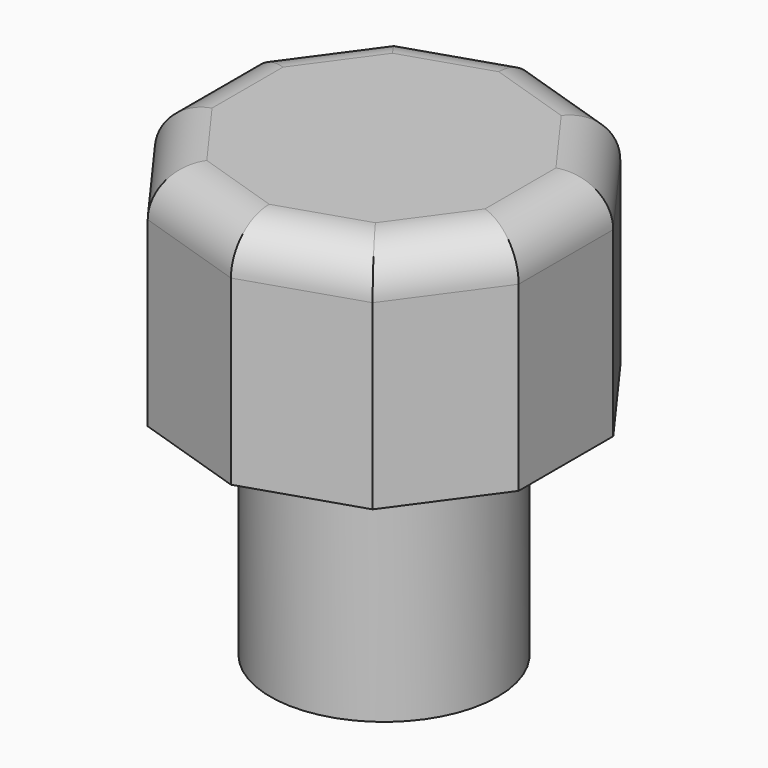
from build123d import *

# Parameters (mm, degrees)
F0_R     = 5
F0_R_2   = 1.6
F1_DEPTH = 10
F3_DEPTH = 8
F5_DEPTH = 2
F6_R     = 1.99999
F8_DEPTH = 3


# Not quite as in the source:
# - a fillet or chamfer is up to 0.001 mm smaller than in the source, because OpenCascade refuses the exact size


with BuildPart() as f1:
    # F0 (on Top) → F1 (new body)
    with BuildSketch(Plane.XY):
        Circle(F0_R)
        Circle(F0_R_2, mode=Mode.SUBTRACT)
    extrude(amount=F1_DEPTH)

    # F2 (on face) → F3 (join)
    with BuildSketch(Plane.XY.offset(10)):
        Polygon((8, -2.5993575699), (8, 2.5993575699), (4.94427191, 6.8052064668), (0, 8.4116977939), (-4.94427191, 6.8052064668), (-8, 2.5993575699), (-8, -2.5993575699), (-4.94427191, -6.8052064668), (0, -8.4116977939), (4.94427191, -6.8052064668), align=None)
        Polygon((0, 3.7527767497), (3.25, 1.8763883749), (3.25, -1.8763883749), (0, -3.7527767497), (-3.25, -1.8763883749), (-3.25, 1.8763883749), align=None, mode=Mode.SUBTRACT)
    extrude(amount=F3_DEPTH)


with BuildPart() as f5:
    # F4 (on face) → F5 (new body)
    with BuildSketch(Plane.XY.offset(18)):
        Polygon((0, 8.4116977939), (-4.94427191, 6.8052064668), (-8, 2.5993575699), (-8, -2.5993575699), (-4.94427191, -6.8052064668), (0, -8.4116977939), (4.94427191, -6.8052064668), (8, -2.5993575699), (8, 2.5993575699), (4.94427191, 6.8052064668), align=None)
    extrude(amount=F5_DEPTH)

    # F6 (radius 2 in the source; OpenCascade refuses exactly that, so slightly less here)
    f6_edges = [f5.edges().sort_by_distance(p)[0] for p in [
        (-2.472136, 7.608452, 20),
        (-6.472136, 4.702282, 20),
        (-8, 0, 20),
        (-6.472136, -4.702282, 20),
        (-2.472136, -7.608452, 20),
        (2.472136, -7.608452, 20),
        (6.472136, -4.702282, 20),
        (8, 0, 20),
        (6.472136, 4.702282, 20),
        (2.472136, 7.608452, 20),
    ]]
    fillet(f6_edges, radius=F6_R)

    # F7 (on face) → F8 (join)
    with BuildSketch(Plane(origin=(0, 0, 18), x_dir=(1, 0, 0), z_dir=(0, 0, -1))):
        Polygon((0, 3.406366662), (-2.9500000639, 1.703183331), (-2.9500000639, -1.703183331), (0, -3.406366662), (2.9500000639, -1.703183331), (2.9500000639, 1.703183331), align=None)
    extrude(amount=F8_DEPTH)


solid = Compound([f1.part, f5.part])
